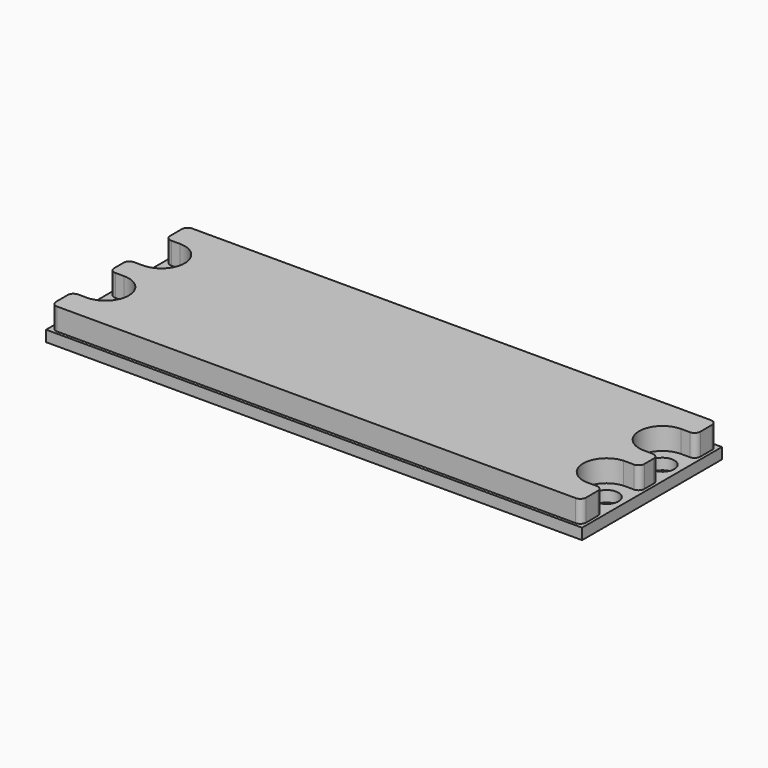
from build123d import *

# Parameters (mm, degrees)
F0_W     = 146.05
F0_H     = 47.625
F0_R     = 3.24
F1_DEPTH = 3
F2_DEPTH = 6
F3_R     = 1.588


# Not quite as in the source:
# - ends of sketch curves that miss each other by under 0.0002 mm in the source are joined


with BuildPart() as f1:
    # F0 (on Top) → F1 (new body)
    with BuildSketch(Plane.XY):
        Rectangle(F0_W, F0_H)
        with Locations((-68.262, -9.5245)):
            Circle(F0_R, mode=Mode.SUBTRACT)
        with Locations((68.262, -9.5245)):
            Circle(F0_R, mode=Mode.SUBTRACT)
        with Locations((-68.262, 9.5245)):
            Circle(F0_R, mode=Mode.SUBTRACT)
        with BuildLine():
            Line((72.225, -15.859485), (72.225, -23.0125))
            Line((72.225, -23.0125), (-72.225, -23.0125))
            Line((-72.225, -23.0125), (-72.225, -15.874133))
            Line((-72.225, -15.874133), (-68.193705, -15.874133))
            ThreePointArc((-68.193705, -15.874133), (-61.912367271, -9.4562050029), (-68.3302949971, -3.174867271))
            Line((-68.3302949971, -3.174867271), (-72.225, -3.174867))
            Line((-72.225, -3.174867), (-72.225, 3.1745))
            Line((-72.225, 3.1745), (-68.262, 3.1745))
            ThreePointArc((-68.262, 3.1745), (-61.912, 9.5245), (-68.262, 15.8745))
            Line((-68.262, 15.8745), (-72.225, 15.8745))
            Line((-72.225, 15.8745), (-72.225, 23.0125))
            Line((-72.225, 23.0125), (72.225, 23.0125))
            Line((72.225, 23.0125), (72.225, 15.8745))
            Line((72.225, 15.8745), (68.262, 15.8745))
            ThreePointArc((68.262, 15.8745), (61.912, 9.5245), (68.262, 3.1745))
            Line((68.262, 3.1745), (72.225, 3.1745))
            Line((72.225, 3.1745), (72.225, -3.189515))
            Line((72.225, -3.189515), (67.825573, -3.189515))
            ThreePointArc((67.825573, -3.189515), (61.9270152731, -9.9609269812), (68.6984269812, -15.8594847269))
            Line((68.6984269812, -15.8594847269), (72.225, -15.859485))
        make_face(mode=Mode.SUBTRACT)
        with Locations((68.262, 9.5245)):
            Circle(F0_R, mode=Mode.SUBTRACT)
        with BuildLine():
            Line((-72.225, -23.0125), (72.225, -23.0125))
            Line((72.225, -23.0125), (72.225, -15.859485))
            Line((72.225, -15.859485), (68.698427, -15.859485))
            ThreePointArc((68.698427, -15.859485), (61.9270152731, -9.9609269812), (67.8255730188, -3.1895152731))
            Line((67.8255730188, -3.1895152731), (72.225, -3.189515))
            Line((72.225, -3.189515), (72.225, 3.1745))
            Line((72.225, 3.1745), (68.262, 3.1745))
            ThreePointArc((68.262, 3.1745), (61.912, 9.5245), (68.262, 15.8745))
            Line((68.262, 15.8745), (72.225, 15.8745))
            Line((72.225, 15.8745), (72.225, 23.0125))
            Line((72.225, 23.0125), (-72.225, 23.0125))
            Line((-72.225, 23.0125), (-72.225, 15.8745))
            Line((-72.225, 15.8745), (-68.262, 15.8745))
            ThreePointArc((-68.262, 15.8745), (-61.912, 9.5245), (-68.262, 3.1745))
            Line((-68.262, 3.1745), (-72.225, 3.1745))
            Line((-72.225, 3.1745), (-72.225, -3.174867))
            Line((-72.225, -3.174867), (-68.330295, -3.174867))
            ThreePointArc((-68.330295, -3.174867), (-61.912367271, -9.4562050029), (-68.1937050029, -15.874132729))
            Line((-68.1937050029, -15.874132729), (-72.225, -15.874133))
            Line((-72.225, -15.874133), (-72.225, -23.0125))
        make_face()
    extrude(amount=-F1_DEPTH)


with BuildPart() as f2:
    # F0 (on Top) → F2 (new body)
    with BuildSketch(Plane.XY):
        with BuildLine():
            Line((-72.225, -23.0125), (72.225, -23.0125))
            Line((72.225, -23.0125), (72.225, -15.859485))
            Line((72.225, -15.859485), (68.698427, -15.859485))
            ThreePointArc((68.698427, -15.859485), (61.9270152731, -9.9609269812), (67.8255730188, -3.1895152731))
            Line((67.8255730188, -3.1895152731), (72.225, -3.189515))
            Line((72.225, -3.189515), (72.225, 3.1745))
            Line((72.225, 3.1745), (68.262, 3.1745))
            ThreePointArc((68.262, 3.1745), (61.912, 9.5245), (68.262, 15.8745))
            Line((68.262, 15.8745), (72.225, 15.8745))
            Line((72.225, 15.8745), (72.225, 23.0125))
            Line((72.225, 23.0125), (-72.225, 23.0125))
            Line((-72.225, 23.0125), (-72.225, 15.8745))
            Line((-72.225, 15.8745), (-68.262, 15.8745))
            ThreePointArc((-68.262, 15.8745), (-61.912, 9.5245), (-68.262, 3.1745))
            Line((-68.262, 3.1745), (-72.225, 3.1745))
            Line((-72.225, 3.1745), (-72.225, -3.174867))
            Line((-72.225, -3.174867), (-68.330295, -3.174867))
            ThreePointArc((-68.330295, -3.174867), (-61.912367271, -9.4562050029), (-68.1937050029, -15.874132729))
            Line((-68.1937050029, -15.874132729), (-72.225, -15.874133))
            Line((-72.225, -15.874133), (-72.225, -23.0125))
        make_face()
    extrude(amount=F2_DEPTH)

    # F3
    f3_edges = [f2.edges().sort_by_distance(p)[0] for p in [
        (-72.225, 23.0125, 3),
        (-72.225, 15.8745, 3),
        (-72.225, 3.1745, 3),
        (-72.225, -3.174867, 3),
        (-72.225, -15.874133, 3),
        (-72.225, -23.0125, 3),
        (72.225, -23.0125, 3),
        (72.225, -15.859485, 3),
        (72.225, -3.189515, 3),
        (72.225, 3.1745, 3),
        (72.225, 23.0125, 3),
        (72.225, 15.8745, 3),
    ]]
    fillet(f3_edges, radius=F3_R)


solid = Compound([f1.part, f2.part])
